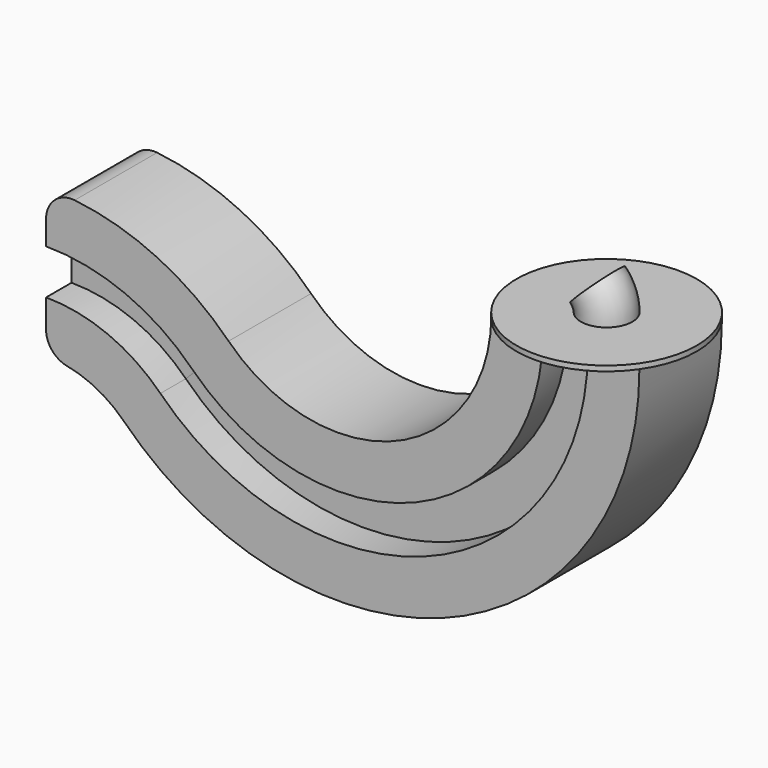
from build123d import *

# Parameters (mm, degrees)
F0_R     = 5
F1_ANGLE = 45
F2_R     = 17.5
F2_R_2   = 5
F3_DEPTH = 1
F5_ANGLE = 135
F7_ANGLE = 45
F8_R     = 5
F9_R     = 5


with BuildPart() as f1:
    # F0 (on Top) → F1 (revolve)
    with BuildSketch(Plane.XY):
        with Locations((17.2625295818, 39.9485491216)):
            Circle(F0_R)
    revolve(axis=Axis((11.3439466804, 38.7977138162, 0), (0, -1, 0)), revolution_arc=F1_ANGLE)

    # F2 (on face) → F3 (join)
    with BuildSketch(Plane(origin=(0, 0, 0), x_dir=(1, 0, 0), z_dir=(0, 0, -1))):
        with Locations((17.2625295818, -39.9485491216)):
            Circle(F2_R)
        with Locations((17.2625295818, -39.9485491216)):
            Circle(F2_R_2, mode=Mode.SUBTRACT)
        with Locations((17.2625295818, -39.9485491216)):
            Circle(F2_R_2)
    extrude(amount=F3_DEPTH)

    # F4 (on face) → F5 (revolve)
    with BuildSketch(Plane(origin=(0, 0, -1), x_dir=(1, 0, 0), z_dir=(0, 0, -1))):
        Polygon((12.9011229654, -29.9485491216), (2.9011229654, -29.9485491216), (2.9011229654, -49.9485491216), (12.9011229654, -49.9485491216), (12.9011229654, -44.1824280606), (21.6239361981, -44.1824280606), (21.6239361981, -49.9485491216), (31.6239361981, -49.9485491216), (31.6239361981, -29.9485491216), (21.6239361981, -29.9485491216), (21.6239361981, -36.1191299331), (12.9011229654, -36.1218505295), align=None)
    revolve(axis=Axis((-26.9732894376, 40.484293364, -1), (0, 1, 0)), revolution_arc=F5_ANGLE)

    # F6 (on face) → F7 (revolve)
    with BuildSketch(Plane(origin=(-12.9866447188, 0, 12.9866447188), x_dir=(0, -1, 0), z_dir=(-0.7071067812, 0, 0.7071067812))):
        Polygon((-36.1218505295, -59.6545150564), (-29.9485491216, -59.6545150564), (-29.9485491216, -49.6545150564), (-49.9485491216, -49.6545150564), (-49.9485491216, -59.6545150564), (-44.1824280606, -59.6545150564), (-44.1824280606, -68.3773282891), (-49.9485491216, -68.3773282891), (-49.9485491216, -78.3773282891), (-29.9485491216, -78.3773282891), (-29.9485491216, -68.3773282891), (-36.1191299331, -68.3773282891), align=None)
    revolve(axis=Axis((-83.5220088064, 42.3686988652, -57.5487193688), (0, -1, 0)), revolution_arc=F7_ANGLE)

    # F8
    f8_edges = [f1.edges().sort_by_distance(p)[0] for p in [
        (-83.522009, 39.948549, -36.173979),
    ]]
    fillet(f8_edges, radius=F8_R)

    # F9
    f9_edges = [f1.edges().sort_by_distance(p)[0] for p in [
        (-83.522009, 39.948549, -7.451166),
    ]]
    fillet(f9_edges, radius=F9_R)


solid = f1.part
